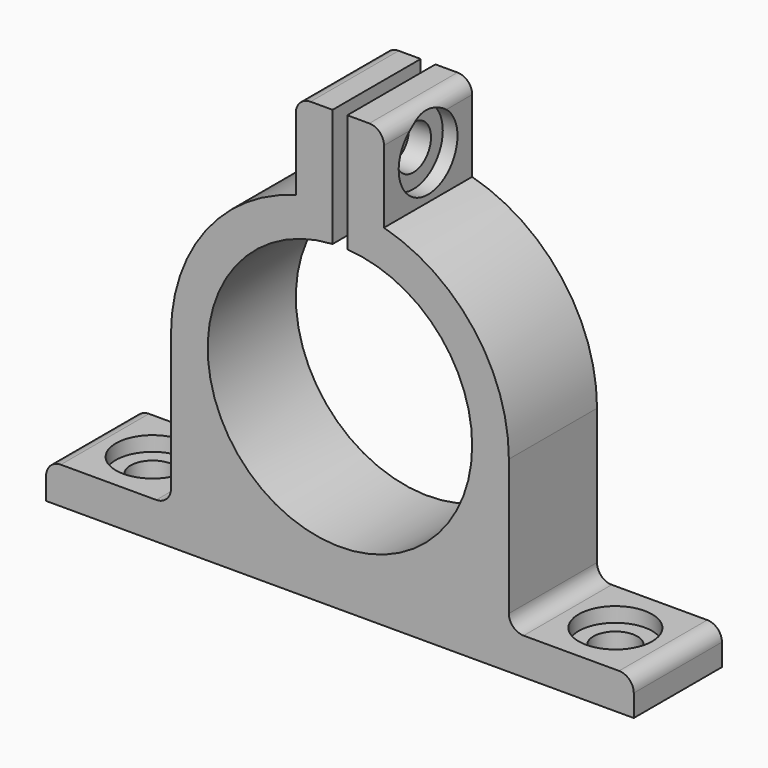
from build123d import *

# Parameters (mm, degrees)
F0_R         = 18
F1_DEPTH     = 15
F3_DEPTH     = 25
F4_R         = 3
F5_DEPTH     = 25
F4_R_2       = 5
F6_DEPTH     = 2
F7_R         = 3
F8_DEPTH     = 25
F7_R_2       = 5
F9_DEPTH     = 2
F10_R        = 3
F11_DEPTH    = 25
F10_R_2      = 5
F12_DEPTH    = 2
F13_T1_DEPTH = 15
F13_T3_DEPTH = 25


# Not quite as in the source:
# - a fillet or chamfer that OpenCascade refuses, or shapes differently, is made with other operations: its cross-section is extruded or revolved along the edge and cut away or added


with BuildPart() as f1:
    # F0 (on Front) → F1 (new body)
    with BuildSketch(Plane.XZ):
        with BuildLine():
            Line((23, -20.5), (10.4283268073, -20.5))
            ThreePointArc((10.4283268073, -20.5), (0, -23), (-10.4283268073, -20.5))
            Line((-10.4283268073, -20.5), (-23, -20.5))
            Line((-23, -20.5), (-40, -20.5))
            Line((-40, -20.5), (-40, -25.5))
            Line((-40, -25.5), (40, -25.5))
            Line((40, -25.5), (40, -20.5))
            Line((40, -20.5), (23, -20.5))
        make_face()
        with BuildLine():
            Line((-23, -20.5), (-10.4283268073, -20.5))
            ThreePointArc((-10.4283268073, -20.5), (-19.606778376, -12.0239029319), (-23, 0))
            Line((-23, 0), (-23, -20.5))
        make_face()
        with BuildLine():
            ThreePointArc((10.4283268073, -20.5), (19.606778376, -12.0239029319), (23, 0))
            ThreePointArc((23, 0), (18.2619823677, 13.9821314541), (6, 22.2036033112))
            Line((6, 22.2036033112), (6, 19.0559069812))
            Line((6, 19.0559069812), (-6, 19.0559069812))
            Line((-6, 19.0559069812), (-6, 22.2036033112))
            ThreePointArc((-6, 22.2036033112), (-18.2619823677, 13.9821314541), (-23, 0))
            ThreePointArc((-23, 0), (-19.606778376, -12.0239029319), (-10.4283268073, -20.5))
            Line((-10.4283268073, -20.5), (10.4283268073, -20.5))
        make_face()
        Circle(F0_R, mode=Mode.SUBTRACT)
        with BuildLine():
            Line((23, -20.5), (23, 0))
            ThreePointArc((23, 0), (19.606778376, -12.0239029319), (10.4283268073, -20.5))
            Line((10.4283268073, -20.5), (23, -20.5))
        make_face()
        with BuildLine():
            ThreePointArc((-10.4283268073, -20.5), (0, -23), (10.4283268073, -20.5))
            Line((10.4283268073, -20.5), (-10.4283268073, -20.5))
        make_face()
        with BuildLine():
            ThreePointArc((-6, 22.2036033112), (0, 23), (6, 22.2036033112))
            Line((6, 22.2036033112), (6, 34.0559069812))
            Line((6, 34.0559069812), (-6, 34.0559069812))
            Line((-6, 34.0559069812), (-6, 22.2036033112))
        make_face()
        with BuildLine():
            Line((6, 19.0559069812), (6, 22.2036033112))
            ThreePointArc((6, 22.2036033112), (0, 23), (-6, 22.2036033112))
            Line((-6, 22.2036033112), (-6, 19.0559069812))
            Line((-6, 19.0559069812), (6, 19.0559069812))
        make_face()
    extrude(amount=F1_DEPTH)

    # F2 (on face) → F3 (cut)
    with BuildSketch(Plane.XZ.offset(15)):
        with BuildLine():
            Line((1, 34.0559069812), (-1, 34.0559069812))
            Line((-1, 34.0559069812), (-1, 17.9722007556))
            ThreePointArc((-1, 17.9722007556), (0, 18), (1, 17.9722007556))
            Line((1, 17.9722007556), (1, 34.0559069812))
        make_face()
    extrude(amount=-F3_DEPTH, mode=Mode.SUBTRACT)

    # F4 (on face) → F5 (cut)
    with BuildSketch(Plane.XY.offset(-20.5)):
        with Locations((31.5, -7.5)):
            Circle(F4_R)
    extrude(amount=-F5_DEPTH, mode=Mode.SUBTRACT)

    # F4 (on face) → F6 (cut)
    with BuildSketch(Plane.XY.offset(-20.5)):
        with Locations((31.5, -7.5)):
            Circle(F4_R_2)
        with Locations((31.5, -7.5)):
            Circle(F4_R, mode=Mode.SUBTRACT)
    extrude(amount=-F6_DEPTH, mode=Mode.SUBTRACT)

    # F7 (on face) → F8 (cut)
    with BuildSketch(Plane.XY.offset(-20.5)):
        with Locations((-31.5, -7.5)):
            Circle(F7_R)
    extrude(amount=-F8_DEPTH, mode=Mode.SUBTRACT)

    # F7 (on face) → F9 (cut)
    with BuildSketch(Plane.XY.offset(-20.5)):
        with Locations((-31.5, -7.5)):
            Circle(F7_R_2)
        with Locations((-31.5, -7.5)):
            Circle(F7_R, mode=Mode.SUBTRACT)
    extrude(amount=-F9_DEPTH, mode=Mode.SUBTRACT)

    # F10 (on face) → F11 (cut)
    with BuildSketch(Plane.YZ.offset(6)):
        with Locations((-7.5, 28.1297551462)):
            Circle(F10_R)
    extrude(amount=-F11_DEPTH, mode=Mode.SUBTRACT)

    # F10 (on face) → F12 (cut)
    with BuildSketch(Plane.YZ.offset(6)):
        with Locations((-7.5, 28.1297551462)):
            Circle(F10_R_2)
        with Locations((-7.5, 28.1297551462)):
            Circle(F10_R, mode=Mode.SUBTRACT)
    extrude(amount=-F12_DEPTH, mode=Mode.SUBTRACT)

    # F13: fillet of radius 2 on 6 edges, made by hand

    # F13_s2 → F13_t1 (join)
    with BuildSketch(Plane.XZ):
        with BuildLine():
            ThreePointArc((25, -20.5), (23.5857864376, -19.9142135624), (23, -18.5))
            Line((23, -18.5), (23, -20.5))
            Line((23, -20.5), (25, -20.5))
        make_face()
        with BuildLine():
            ThreePointArc((-25, -20.5), (-23.5857864376, -19.9142135624), (-23, -18.5))
            Line((-23, -18.5), (-23, -20.5))
            Line((-23, -20.5), (-25, -20.5))
        make_face()
    extrude(amount=F13_T1_DEPTH)

    # F13_s4 → F13_t3 (cut)
    with BuildSketch(Plane.XZ.offset(-5)):
        with BuildLine():
            ThreePointArc((-6, 32.0559069812), (-5.4142135624, 33.4701205436), (-4, 34.0559069812))
            Line((-4, 34.0559069812), (-6, 34.0559069812))
            Line((-6, 34.0559069812), (-6, 32.0559069812))
        make_face()
        with BuildLine():
            ThreePointArc((4, 34.0559069812), (5.4142135624, 33.4701205436), (6, 32.0559069812))
            Line((6, 32.0559069812), (6, 34.0559069812))
            Line((6, 34.0559069812), (4, 34.0559069812))
        make_face()
        with BuildLine():
            ThreePointArc((38, -20.5), (39.4142135624, -21.0857864376), (40, -22.5))
            Line((40, -22.5), (40, -20.5))
            Line((40, -20.5), (38, -20.5))
        make_face()
        with BuildLine():
            ThreePointArc((-40, -22.5), (-39.4142135624, -21.0857864376), (-38, -20.5))
            Line((-38, -20.5), (-40, -20.5))
            Line((-40, -20.5), (-40, -22.5))
        make_face()
    extrude(amount=F13_T3_DEPTH, mode=Mode.SUBTRACT)


solid = f1.part
